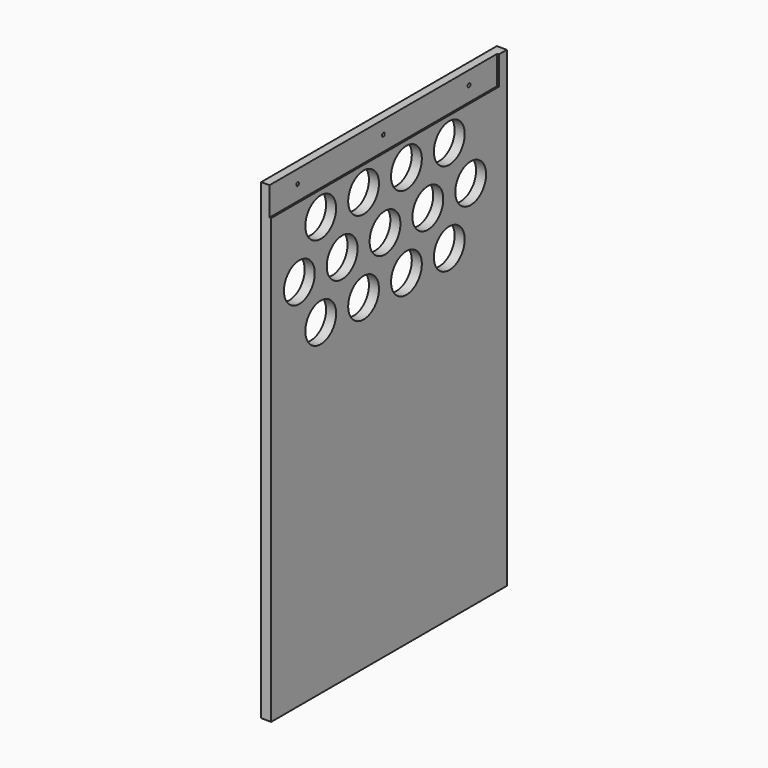
from build123d import *

# Parameters (mm, degrees)
F0_W     = 19.05
F0_H     = 337.82
F1_DEPTH = 539.75
F2_R     = 36.5125
F3_DEPTH = 25.4
F4_DEPTH = 557.53
F5_DEPTH = 19.05
F6_W     = 3.175
F6_H     = 53.975
F7_DEPTH = 539.75
F9_D     = 6.5278


# Not quite as in the source:
# - a feature names something its author has since deleted; it is built from what else it names


with BuildPart() as f1:
    # F0 (on Front) → F1 (new body)
    with BuildSketch(Plane.XZ):
        Rectangle(F0_W, F0_H)
    extrude(amount=F1_DEPTH)

    # F2 (on face) → F3 (cut)
    with BuildSketch(Plane.YZ.offset(9.525)):
        with Locations((-269.875, -19.05)):
            Circle(F2_R)
        with Locations((-320.6515127996, 68.8975)):
            Circle(F2_R)
        with Locations((-219.0515127996, 68.8975)):
            Circle(F2_R)
        with Locations((-168.275, -19.05)):
            Circle(F2_R)
        with Locations((-117.4515127996, 68.8975)):
            Circle(F2_R)
        with Locations((-66.675, -19.05)):
            Circle(F2_R)
        with Locations((-371.475, -19.05)):
            Circle(F2_R)
        with Locations((-422.2984872004, 68.8975)):
            Circle(F2_R)
        with Locations((-473.075, -19.05)):
            Circle(F2_R)
        with Locations((-422.2984872004, -106.9975)):
            Circle(F2_R)
        with Locations((-320.6515127996, -106.9975)):
            Circle(F2_R)
        with Locations((-219.0515127996, -106.9975)):
            Circle(F2_R)
        with Locations((-117.4515127996, -106.9975)):
            Circle(F2_R)
    extrude(amount=-F3_DEPTH, mode=Mode.SUBTRACT)

    # F4 (add): a face of the model
    f4_faces = [f1.faces().sort_by_distance(p)[0] for p in [
        (0, -269.875, -168.91),
    ]]
    extrude(f4_faces, amount=F4_DEPTH)

    # F5 (add): a face of the model
    f5_faces = [f1.faces().sort_by_distance(p)[0] for p in [
        (0, 0, -278.765),
    ]]
    extrude(f5_faces, amount=F5_DEPTH)

    # F6 (on face) → F7 (cut, through all)
    with BuildSketch(Plane.XZ.offset(539.75)):
        with Locations((7.9375, 141.9225)):
            Rectangle(F6_W, F6_H)
    extrude(amount=-F7_DEPTH, mode=Mode.SUBTRACT)

    # F9 (through all)
    with Locations(Plane(origin=(-9.525, 0, 0), x_dir=(0, -1, 0), z_dir=(-1, 0, 0))):
        with Locations((66.675, 143.51), (269.875, 143.51), (473.075, 143.51)):
            Hole(F9_D / 2)


solid = f1.part
